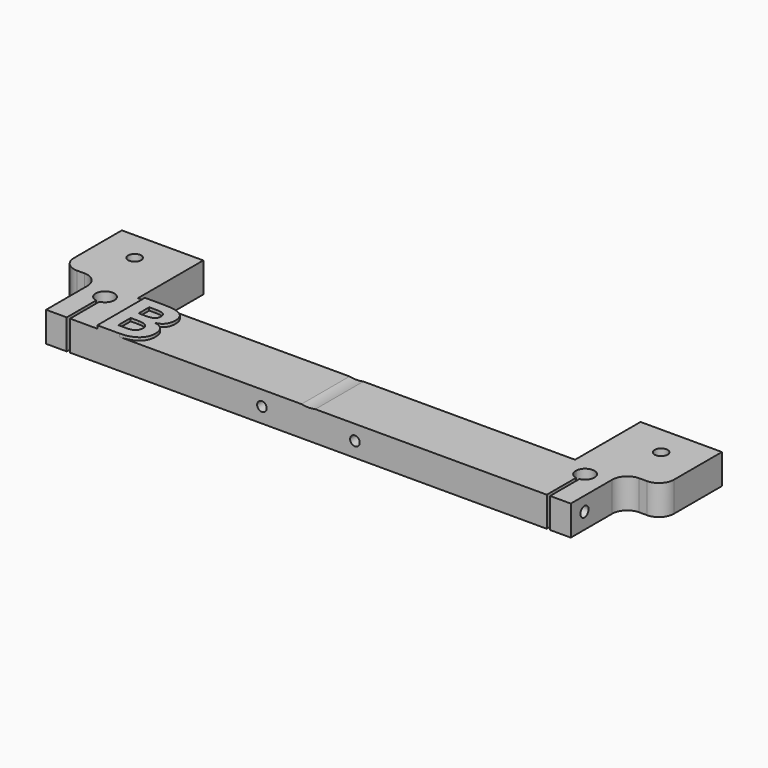
from build123d import *

# Parameters (mm, degrees)
F1_DEPTH      = 10
F2_R          = 1.6
F2_R_2        = 10.75
F3_DEPTH      = 47.2759499461
F4_R          = 2.175
F5_DEPTH      = 10.001
F6_R          = 5
F7_R          = 5
F8_R          = 1.4
F9_DEPTH      = 18
F8_R_2        = 1.7
F10_DEPTH     = 6.8896186928
F12_TEXT_SIZE = 27.7777777778
F13_DEPTH     = 1


# Not quite as in the source:
# - Text() gives the source's letters only with a copy of the font that has no kerning and outlines rounded to 1/6400 em; it was checked with that copy


with BuildPart() as f1:
    # F0 (on Top) → F1 (new body)
    with BuildSketch(Plane.XY):
        Polygon((-87.4418646097, -13.8158900663), (0, -13.8158900663), (0, 6.1841099337), (-72.8655805642, 6.1841099337), (-72.8655805642, 33.4590598798), (-100, 33.4590598798), (-100, 8.4590598798), (-87.4418646097, 8.4590598798), align=None)
    extrude(amount=F1_DEPTH)

    # F2 (on face) → F3 (cut, through all)
    with BuildSketch(Plane.XZ.offset(13.8158900663)):
        with Locations((-15.5, 5)):
            Circle(F2_R)
        with Locations((0, 20.5)):
            Circle(F2_R_2)
    extrude(amount=-F3_DEPTH, mode=Mode.SUBTRACT)

    # F4 (on face) → F5 (cut, through all)
    with BuildSketch(Plane.XY.offset(10)):
        with BuildLine():
            ThreePointArc((-79.446754083, -1.5911727269), (-77.6203926435, -0.5277639243), (-76.9, 1.4590598798))
            ThreePointArc((-76.9, 1.4590598798), (-81.9868238041, 3.8386672364), (-80.553245917, -1.5911727269))
            Line((-80.553245917, -1.5911727269), (-80.553245917, -0.7115720073))
            Line((-80.553245917, -0.7115720073), (-79.446754083, -0.7115720073))
            Line((-79.446754083, -0.7115720073), (-79.446754083, -1.5911727269))
        make_face()
        with BuildLine():
            Line((-80.553245917, -0.7115720073), (-80.553245917, -1.5911727269))
            ThreePointArc((-80.553245917, -1.5911727269), (-80, -1.6409401202), (-79.446754083, -1.5911727269))
            Line((-79.446754083, -1.5911727269), (-79.446754083, -0.7115720073))
            Line((-79.446754083, -0.7115720073), (-80.553245917, -0.7115720073))
        make_face()
        with BuildLine():
            ThreePointArc((-79.446754083, -1.5911727269), (-80, -1.6409401202), (-80.553245917, -1.5911727269))
            Line((-80.553245917, -1.5911727269), (-80.553245917, -13.8158900663))
            Line((-80.553245917, -13.8158900663), (-79.446754083, -13.8158900663))
            Line((-79.446754083, -13.8158900663), (-79.446754083, -1.5911727269))
        make_face()
        with Locations((-87.7414673567, 23.4590598798)):
            Circle(F4_R)
    extrude(amount=-F5_DEPTH, mode=Mode.SUBTRACT)

    # F6
    f6_edges = [f1.edges().sort_by_distance(p)[0] for p in [
        (-100, 8.45906, 5),
    ]]
    fillet(f6_edges, radius=F6_R)

    # F7
    f7_edges = [f1.edges().sort_by_distance(p)[0] for p in [
        (-87.441865, 8.45906, 5),
    ]]
    fillet(f7_edges, radius=F7_R)

    # F8 (on face) → F9 (cut)
    with BuildSketch(Plane(origin=(-87.4418646097, 0, 0), x_dir=(0, -1, 0), z_dir=(-1, 0, 0))):
        with Locations((8.1005264074, 5.3087547421)):
            Circle(F8_R)
    extrude(amount=-F9_DEPTH, mode=Mode.SUBTRACT)

    # F8 (on face) → F10 (cut, through all)
    with BuildSketch(Plane(origin=(-87.4418646097, 0, 0), x_dir=(0, -1, 0), z_dir=(-1, 0, 0))):
        with Locations((8.1005264074, 5.3087547421)):
            Circle(F8_R_2)
        with Locations((8.1005264074, 5.3087547421)):
            Circle(F8_R, mode=Mode.SUBTRACT)
        with Locations((8.1005264074, 5.3087547421)):
            Circle(F8_R)
    extrude(amount=-F10_DEPTH, mode=Mode.SUBTRACT)

    # F11: F1 across plane


with BuildPart() as f1_1:
    add(f1.part)
    add(f1.part.mirror(Plane.YZ))

    # F12 (on face) → F13 (join)
    with BuildSketch(Plane.XY.offset(10)):
        with Locations((-72.8655805642, -13.8158900663)):
            Text('B', F12_TEXT_SIZE, font='Open Sans', font_style=FontStyle.BOLD, text_align=(TextAlign.LEFT, TextAlign.BOTTOM))
    extrude(amount=F13_DEPTH)


solid = f1_1.part
